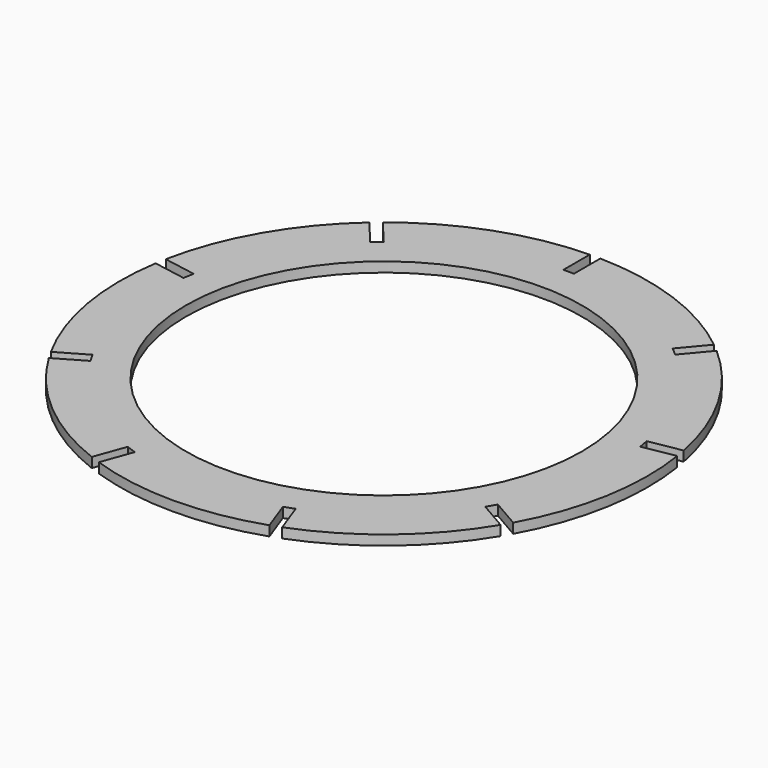
from build123d import *

# Parameters (mm, degrees)
F0_R            = 80
F0_R_2          = 60
F1_DEPTH        = 3
F2_W            = 3.2
F2_H            = 10
F3_DEPTH        = 25
F3_COPIES_COUNT = 9


# Not quite as in the source:
# - a pattern or mirror of a feature is missing from the dataset's text; its kind, count and spacing are read off the source's solid


with BuildPart() as f1:
    # F0 (on Top) → F1 (new body)
    with BuildSketch(Plane.XY):
        Circle(F0_R)
        Circle(F0_R_2, mode=Mode.SUBTRACT)
    extrude(amount=F1_DEPTH)

    # F2 (on face) → F3 (cut)
    with BuildSketch(Plane.XY.offset(3)):
        with Locations((0, 75)):
            Rectangle(F2_W, F2_H)
    f3 = extrude(amount=-F3_DEPTH, mode=Mode.SUBTRACT)

    # F3_copies: F3 ×9 about axis
    f3_copies_axis = Axis((0, 0, 0), (0, 0, 1))
    for i in range(1, F3_COPIES_COUNT):
        add(f3.rotate(f3_copies_axis, i * 360 / F3_COPIES_COUNT), mode=Mode.SUBTRACT)


solid = f1.part
